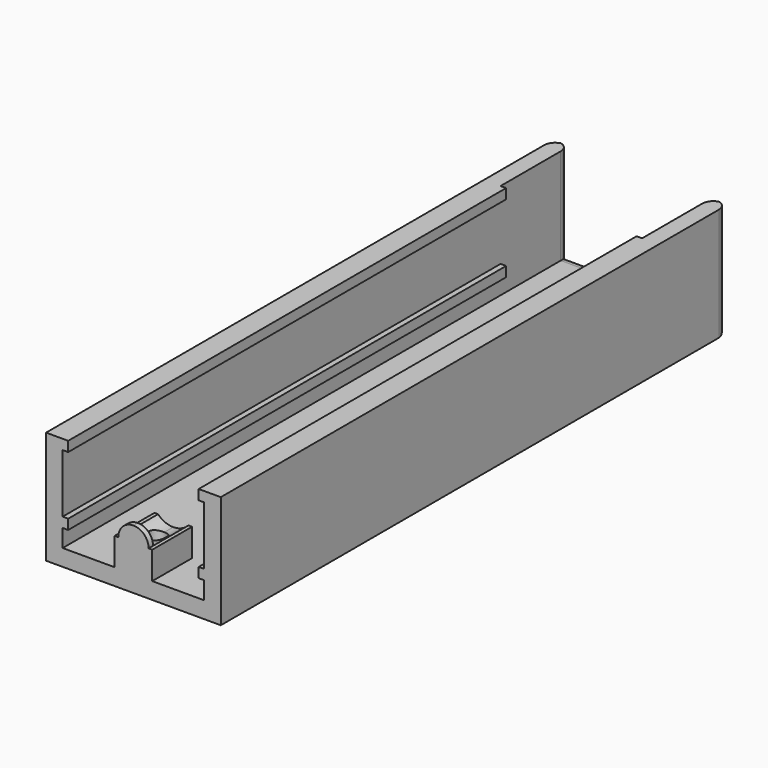
from build123d import *

# Parameters (mm, degrees)
F1_DEPTH      = 114.6
F3_DEPTH      = 105.6
F5_DEPTH      = 8
F6_R          = 1.5
F7_DEPTH      = 20.401
F8_W          = 1
F8_H          = 1.8
F9_DEPTH      = 15.6
F10_T1_DEPTH  = 22.4
F10_T3_DEPTH  = 30.4
F10_T5_DEPTH  = 25.6
F10_T7_DEPTH  = 41.6
F10_T13_DEPTH = 30.6
F10_T17_DEPTH = 27.4
F10_T24_DEPTH = 30.6
F10_T28_DEPTH = 27.4


# Not quite as in the source:
# - a fillet or chamfer that OpenCascade refuses, or shapes differently, is made with other operations: its cross-section is extruded or revolved along the edge and cut away or added


with BuildPart() as f1:
    # F0 (on Front) → F1 (new body)
    with BuildSketch(Plane.XZ):
        Polygon((-15.8, 0), (0, 0), (15.8, 0), (15.8, 20.4), (11.8, 20.4), (11.8, 18.6), (12.8, 18.6), (12.8, 8), (11.8, 8), (11.8, 6.2), (12.8, 6.2), (12.8, 3), (3.4, 3), (3.4, 8), (2.75, 8), (0, 8), (-2.75, 8), (-3.4, 8), (-3.4, 3), (-12.8, 3), (-12.8, 6.2), (-11.8, 6.2), (-11.8, 8), (-12.8, 8), (-12.8, 18.6), (-11.8, 18.6), (-11.8, 20.4), (-15.8, 20.4), align=None)
        with BuildLine():
            ThreePointArc((0, 10.75), (-1.9445436483, 9.9445436483), (-2.75, 8))
            Line((-2.75, 8), (0, 8))
            Line((0, 8), (0, 10.75))
        make_face()
        with BuildLine():
            Line((0, 8), (2.75, 8))
            ThreePointArc((2.75, 8), (1.9445436483, 9.9445436483), (0, 10.75))
            Line((0, 10.75), (0, 8))
        make_face()
    extrude(amount=F1_DEPTH)

    # F2 (on face) → F3 (cut)
    with BuildSketch(Plane(origin=(0, 0, 0), x_dir=(-1, 0, 0), z_dir=(0, 1, 0))):
        with BuildLine():
            Line((-3.4, 8), (-3.4, 3))
            Line((-3.4, 3), (3.4, 3))
            Line((3.4, 3), (3.4, 8))
            Line((3.4, 8), (2.75, 8))
            ThreePointArc((2.75, 8), (0, 10.75), (-2.75, 8))
            Line((-2.75, 8), (-3.4, 8))
        make_face()
    extrude(amount=-F3_DEPTH, mode=Mode.SUBTRACT)

    # F4 (on face) → F5 (cut)
    with BuildSketch(Plane(origin=(0, -105.6, 0), x_dir=(-1, 0, 0), z_dir=(0, 1, 0))):
        with BuildLine():
            ThreePointArc((2.75, 8), (0, 10.75), (-2.75, 8))
            ThreePointArc((-2.75, 8), (-1.4940831044, 7.1353558864), (0, 6.8309673695))
            ThreePointArc((0, 6.8309673695), (1.4940831044, 7.1353558864), (2.75, 8))
        make_face()
    extrude(amount=-F5_DEPTH, mode=Mode.SUBTRACT)

    # F6 (on face) → F7 (cut, through all)
    with BuildSketch(Plane(origin=(0, 0, 0), x_dir=(1, 0, 0), z_dir=(0, 0, -1))):
        with Locations((0, 109.1)):
            Circle(F6_R)
    extrude(amount=-F7_DEPTH, mode=Mode.SUBTRACT)

    # F8 (on face) → F9 (cut)
    with BuildSketch(Plane(origin=(0, 0, 0), x_dir=(-1, 0, 0), z_dir=(0, 1, 0))):
        with Locations((-12.3, 19.5)):
            Rectangle(F8_W, F8_H)
        with Locations((-12.3, 7.1)):
            Rectangle(F8_W, F8_H)
        with Locations((12.3, 7.1)):
            Rectangle(F8_W, F8_H)
        with Locations((12.3, 19.5)):
            Rectangle(F8_W, F8_H)
    extrude(amount=-F9_DEPTH, mode=Mode.SUBTRACT)

    # F10: fillet of radius 2 on 6 edges, made by hand

    # F10_s2 → F10_t1 (cut)
    with BuildSketch(Plane.XY.offset(3)):
        with BuildLine():
            ThreePointArc((12.8, -2), (13.3857864376, -0.5857864376), (14.8, 0))
            Line((14.8, 0), (12.8, 0))
            Line((12.8, 0), (12.8, -2))
        make_face()
        with BuildLine():
            ThreePointArc((-12.8, -2), (-13.3857864376, -0.5857864376), (-14.8, 0))
            Line((-14.8, 0), (-12.8, 0))
            Line((-12.8, 0), (-12.8, -2))
        make_face()
    extrude(amount=F10_T1_DEPTH, mode=Mode.SUBTRACT)

    # F10_s4 → F10_t3 (cut)
    with BuildSketch(Plane.XY.offset(-5)):
        with BuildLine():
            ThreePointArc((15.8, -2), (15.2142135624, -0.5857864376), (13.8, 0))
            Line((13.8, 0), (15.8, 0))
            Line((15.8, 0), (15.8, -2))
        make_face()
        with BuildLine():
            ThreePointArc((-13.8, 0), (-15.2142135624, -0.5857864376), (-15.8, -2))
            Line((-15.8, -2), (-15.8, 0))
            Line((-15.8, 0), (-13.8, 0))
        make_face()
    extrude(amount=F10_T3_DEPTH, mode=Mode.SUBTRACT)

    # F10_s6 → F10_t5 (cut)
    with BuildSketch(Plane.YZ.offset(-12.8)):
        with BuildLine():
            ThreePointArc((-2, 3), (-0.5857864376, 2.4142135624), (0, 1))
            Line((0, 1), (0, 3))
            Line((0, 3), (-2, 3))
        make_face()
    extrude(amount=F10_T5_DEPTH, mode=Mode.SUBTRACT)

    # F10_s8 → F10_t7 (cut)
    with BuildSketch(Plane.YZ.offset(-20.8)):
        with BuildLine():
            ThreePointArc((-2, 0), (-0.5857864376, 0.5857864376), (0, 2))
            Line((0, 2), (0, 0))
            Line((0, 0), (-2, 0))
        make_face()
    extrude(amount=F10_T7_DEPTH, mode=Mode.SUBTRACT)


with BuildPart() as f10_tool11:
    # F10_s12 → F10_t13 (new body)
    with BuildSketch(Plane.YZ.offset(-12.8)):
        with BuildLine():
            ThreePointArc((-2, 3), (-0.5857864376, 2.4142135624), (0, 1))
            Line((0, 1), (0, 3))
            Line((0, 3), (-2, 3))
        make_face()
    extrude(amount=F10_T13_DEPTH)

    split(bisect_by=Plane.YZ.offset(12.8), keep=Keep.TOP)


with BuildPart() as f10_tool15:
    # F10_s16 → F10_t17 (new body)
    with BuildSketch(Plane.XY.offset(-2)):
        with BuildLine():
            ThreePointArc((12.8, -2), (13.3857864376, -0.5857864376), (14.8, 0))
            Line((14.8, 0), (12.8, 0))
            Line((12.8, 0), (12.8, -2))
        make_face()
    extrude(amount=F10_T17_DEPTH)

    split(bisect_by=Plane.XY.offset(3), keep=Keep.BOTTOM)


with BuildPart() as f10_tool11_1:
    add(f10_tool11.part)

    # F10_t19: intersect F10_tool15
    add(f10_tool15.part, mode=Mode.INTERSECT)


with BuildPart() as f1_1:
    add(f1.part)

    # F10_t9: cut F10_tool11
    add(f10_tool11_1.part, mode=Mode.SUBTRACT)


with BuildPart() as f10_tool22:
    # F10_s23 → F10_t24 (new body)
    with BuildSketch(Plane.YZ.offset(-17.8)):
        with BuildLine():
            ThreePointArc((-2, 3), (-0.5857864376, 2.4142135624), (0, 1))
            Line((0, 1), (0, 3))
            Line((0, 3), (-2, 3))
        make_face()
    extrude(amount=F10_T24_DEPTH)

    split(bisect_by=Plane.YZ.offset(-12.8), keep=Keep.BOTTOM)


with BuildPart() as f10_tool26:
    # F10_s27 → F10_t28 (new body)
    with BuildSketch(Plane.XY.offset(25.4)):
        with BuildLine():
            ThreePointArc((-12.8, -2), (-13.3857864376, -0.5857864376), (-14.8, 0))
            Line((-14.8, 0), (-12.8, 0))
            Line((-12.8, 0), (-12.8, -2))
        make_face()
    extrude(amount=-F10_T28_DEPTH)

    split(bisect_by=Plane.XY.offset(3), keep=Keep.BOTTOM)


with BuildPart() as f10_tool22_1:
    add(f10_tool22.part)

    # F10_t30: intersect F10_tool26
    add(f10_tool26.part, mode=Mode.INTERSECT)


with BuildPart() as f1_2:
    add(f1_1.part)

    # F10_t20: cut F10_tool22
    add(f10_tool22_1.part, mode=Mode.SUBTRACT)


solid = f1_2.part
